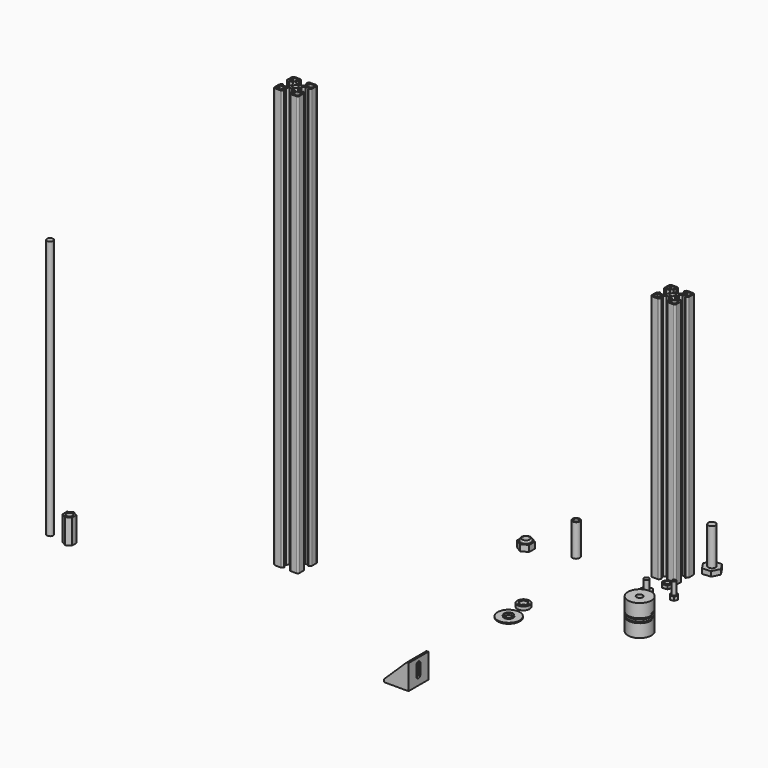
from build123d import *

# Parameters (mm, degrees)
F1_R      = 2.1
F2_DEPTH  = 340
F3_R      = 3
F4_DEPTH  = 34
F5_DEPTH  = 4
F6_R      = 3
F6_R_2    = 2
F7_DEPTH  = 26
F8_R      = 2
F9_DEPTH  = 3
F10_DEPTH = 11
F12_DEPTH = 25
F13_DEPTH = 25
F14_DEPTH = 10.04921
F15_START = 11.79412
F15_DEPTH = 1.02436
F16_START = 13.17687
F16_DEPTH = 1.01812
F17_START = 14.75436
F17_DEPTH = 1.27008
F18_START = 10.61296
F18_DEPTH = 0.97243
F0_R      = 2.1
F20_DEPTH = 200
F21_R     = 2.5
F22_DEPTH = 210
F23_DEPTH = 20
F24_W     = 18.5
F24_H     = 20
F25_DEPTH = 2
F26_W     = 20
F26_H     = 18
F26_H_2   = 2
F27_DEPTH = 1.5
F19_R     = 4
F19_R_2   = 3
F29_DEPTH = 3
F19_R_3   = 5
F19_R_4   = 4.5
F30_DEPTH = 2.8
F31_DEPTH = 0.2
F19_R_5   = 3.75
F19_R_6   = 3.05
F32_DEPTH = 1.5
F19_R_7   = 9
F19_R_8   = 6.5
F33_DEPTH = 0.8
F35_DEPTH = 2
F37_DEPTH = 2
F38_DEPTH = 3
F39_DEPTH = 15
F40_DEPTH = 3
F41_R     = 0.5
F8_R_2    = 1.5
F42_DEPTH = 3
F43_DEPTH = 13
F44_R     = 4.0653248117
F44_R_2   = 3
F45_DEPTH = 5
F46_DEPTH = 7
F47_R     = 1


# Not quite as in the source:
# - ends of sketch curves that miss each other by under 0.0002 mm in the source are joined
# - a feature of the source that left no trace in its solid (it failed there, or was rolled back) is left out


with BuildPart() as f2:
    # F1 (on Top) → F2 (new body)
    with BuildSketch(Plane.XY):
        with BuildLine():
            ThreePointArc((-76.0568475723, -59.3990511647), (-75.9967122677, -59.7013714029), (-75.8254614295, -59.9576660218))
            Line((-75.8254614295, -59.9576660218), (-74.5429985723, -61.2401291647))
            ThreePointArc((-74.5429985723, -61.2401291647), (-74.3297821853, -61.2853778355), (-74.2018372512, -61.1089161811))
            Line((-74.2018372512, -61.1089161811), (-74.2018375723, -60.0487081647))
            Line((-74.2018375723, -60.0487081647), (-71.0852305723, -60.0487081647))
            Line((-71.0852305723, -60.0487081647), (-69.4568475723, -61.6826121647))
            Line((-69.4568475723, -61.6826121647), (-69.4568475723, -63.2678111647))
            Line((-69.4568475723, -63.2678111647), (-69.0759505723, -63.6487081647))
            Line((-69.0759505723, -63.6487081647), (-69.4568475723, -64.0296051647))
            Line((-69.4568475723, -64.0296051647), (-69.4568475723, -65.6148041647))
            Line((-69.4568475723, -65.6148041647), (-71.0852305723, -67.2487081647))
            Line((-71.0852305723, -67.2487081647), (-74.2018375723, -67.2487081647))
            Line((-74.2018375723, -67.2487081647), (-74.2018375723, -66.1885001647))
            ThreePointArc((-74.2018375723, -66.1885001647), (-74.3297821853, -66.0120384939), (-74.5429984286, -66.0572873085))
            Line((-74.5429984286, -66.0572873085), (-75.8254615723, -67.3397501647))
            ThreePointArc((-75.8254615723, -67.3397501647), (-75.9967122677, -67.5960449265), (-76.0568475723, -67.8983651647))
            Line((-76.0568475723, -67.8983651647), (-76.0568475723, -72.2296051647))
            ThreePointArc((-76.0568475723, -72.2296051647), (-75.6261258719, -73.2058338929), (-74.6553495591, -73.6487079596))
            Line((-74.6553495591, -73.6487079596), (-70.0996785723, -73.6487081647))
            ThreePointArc((-70.0996785723, -73.6487081647), (-69.7935318264, -73.5878117907), (-69.5339931474, -73.4143935896))
            Line((-69.5339931474, -73.4143935896), (-68.4300705723, -72.3104711647))
            ThreePointArc((-68.4300705723, -72.3104711647), (-68.3758776892, -72.0380233066), (-68.6068475723, -71.8836941647))
            Line((-68.6068475723, -71.8836941647), (-69.6568475723, -71.8836941647))
            Line((-69.6568475723, -71.8836941647), (-69.6568475723, -68.6836941647))
            Line((-69.6568475723, -68.6836941647), (-68.0622535723, -67.0836941647))
            Line((-68.0622535723, -67.0836941647), (-66.3568475723, -67.0836941647))
            Line((-66.3568475723, -67.0836941647), (-66.0568475723, -66.8237411647))
            Line((-66.0568475723, -66.8237411647), (-65.7568475723, -67.0836941647))
            Line((-65.7568475723, -67.0836941647), (-64.0514415723, -67.0836941647))
            Line((-64.0514415723, -67.0836941647), (-62.4568475723, -68.6836941647))
            Line((-62.4568475723, -68.6836941647), (-62.4568475723, -71.8836941647))
            Line((-62.4568475723, -71.8836941647), (-63.5068475723, -71.8836941647))
            ThreePointArc((-63.5068475723, -71.8836941647), (-63.7378174555, -72.0380233066), (-63.6836242676, -72.31047086))
            Line((-63.6836242676, -72.31047086), (-62.5797015723, -73.4143931647))
            ThreePointArc((-62.5797015723, -73.4143931647), (-62.3201633182, -73.5878117907), (-62.0140165723, -73.6487081647))
            Line((-62.0140165723, -73.6487081647), (-57.4583455723, -73.6487081647))
            ThreePointArc((-57.4583455723, -73.6487081647), (-56.4875692727, -73.2058338929), (-56.0568470783, -72.2296051903))
            Line((-56.0568470783, -72.2296051903), (-56.0568475723, -67.8983651647))
            ThreePointArc((-56.0568475723, -67.8983651647), (-56.1169828769, -67.5960449265), (-56.2882337152, -67.3397503076))
            Line((-56.2882337152, -67.3397503076), (-57.5706965723, -66.0572871647))
            ThreePointArc((-57.5706965723, -66.0572871647), (-57.7839129594, -66.0120384939), (-57.9118578934, -66.1885001483))
            Line((-57.9118578934, -66.1885001483), (-57.9118575723, -67.2487081647))
            Line((-57.9118575723, -67.2487081647), (-61.0284645723, -67.2487081647))
            Line((-61.0284645723, -67.2487081647), (-62.6568475723, -65.6148041647))
            Line((-62.6568475723, -65.6148041647), (-62.6568475723, -64.0296051647))
            Line((-62.6568475723, -64.0296051647), (-63.0377445723, -63.6487081647))
            Line((-63.0377445723, -63.6487081647), (-62.6568475723, -63.2678111647))
            Line((-62.6568475723, -63.2678111647), (-62.6568475723, -61.6826121647))
            Line((-62.6568475723, -61.6826121647), (-61.0284645723, -60.0487081647))
            Line((-61.0284645723, -60.0487081647), (-57.9118575723, -60.0487081647))
            Line((-57.9118575723, -60.0487081647), (-57.9118575723, -61.1089161647))
            ThreePointArc((-57.9118575723, -61.1089161647), (-57.7839129594, -61.2853778355), (-57.5706967161, -61.2401290209))
            Line((-57.5706967161, -61.2401290209), (-56.2882335723, -59.9576661647))
            ThreePointArc((-56.2882335723, -59.9576661647), (-56.1169828769, -59.7013714029), (-56.0568475723, -59.3990511647))
            Line((-56.0568475723, -59.3990511647), (-56.0568475723, -55.0678111647))
            ThreePointArc((-56.0568475723, -55.0678111647), (-56.4875692727, -54.0915824365), (-57.4583455855, -53.6487083698))
            Line((-57.4583455855, -53.6487083698), (-62.0140165723, -53.6487081647))
            ThreePointArc((-62.0140165723, -53.6487081647), (-62.3201633182, -53.7096045387), (-62.5797019973, -53.8830227397))
            Line((-62.5797019973, -53.8830227397), (-63.6836245723, -54.9869451647))
            ThreePointArc((-63.6836245723, -54.9869451647), (-63.7378174555, -55.2593930228), (-63.5068475723, -55.4137221647))
            Line((-63.5068475723, -55.4137221647), (-62.4568475723, -55.4137221647))
            Line((-62.4568475723, -55.4137221647), (-62.4568475723, -58.6137221647))
            Line((-62.4568475723, -58.6137221647), (-64.0514415723, -60.2137221647))
            Line((-64.0514415723, -60.2137221647), (-65.7568475723, -60.2137221647))
            Line((-65.7568475723, -60.2137221647), (-66.0568475723, -60.4736751647))
            Line((-66.0568475723, -60.4736751647), (-66.3568475723, -60.2137221647))
            Line((-66.3568475723, -60.2137221647), (-68.0622535723, -60.2137221647))
            Line((-68.0622535723, -60.2137221647), (-69.6568475723, -58.6137221647))
            Line((-69.6568475723, -58.6137221647), (-69.6568475723, -55.4137221647))
            Line((-69.6568475723, -55.4137221647), (-68.6068475723, -55.4137221647))
            ThreePointArc((-68.6068475723, -55.4137221647), (-68.3758776892, -55.2593930228), (-68.430070877, -54.9869454694))
            Line((-68.430070877, -54.9869454694), (-69.5339935723, -53.8830231647))
            ThreePointArc((-69.5339935723, -53.8830231647), (-69.7935318264, -53.7096045387), (-70.0996785723, -53.6487081647))
            Line((-70.0996785723, -53.6487081647), (-74.6553495723, -53.6487081647))
            ThreePointArc((-74.6553495723, -53.6487081647), (-75.6261258719, -54.0915824365), (-76.0568480663, -55.067811139))
            Line((-76.0568480663, -55.067811139), (-76.0568475723, -59.3990511647))
        make_face()
        with BuildLine():
            Line((-74.8568475723, -72.0296051647), (-74.8568475723, -69.0296051647))
            ThreePointArc((-74.8568475723, -69.0296051647), (-74.7726451834, -68.6531880416), (-74.4455855613, -68.4487082319))
            Line((-74.4455855613, -68.4487082319), (-71.4455855723, -68.4487081647))
            ThreePointArc((-71.4455855723, -68.4487081647), (-70.9974332481, -68.5832975965), (-70.8568471738, -69.0296052379))
            Line((-70.8568471738, -69.0296052379), (-70.8568475723, -72.0296051647))
            ThreePointArc((-70.8568475723, -72.0296051647), (-71.0651110441, -72.369091567), (-71.4553494884, -72.4487077678))
            Line((-71.4553494884, -72.4487077678), (-74.4553495723, -72.4487081647))
            ThreePointArc((-74.4553495723, -72.4487081647), (-74.7231318194, -72.303374032), (-74.8568475723, -72.0296051647))
        make_face(mode=Mode.SUBTRACT)
        with BuildLine():
            ThreePointArc((-61.2568479709, -69.0296052379), (-61.1162618966, -68.5832975965), (-60.6681095129, -68.4487078641))
            Line((-60.6681095129, -68.4487078641), (-57.6681095723, -68.4487081647))
            ThreePointArc((-57.6681095723, -68.4487081647), (-57.3410499613, -68.6531880416), (-57.2568472544, -69.0296052212))
            Line((-57.2568472544, -69.0296052212), (-57.2568475723, -72.0296051647))
            ThreePointArc((-57.2568475723, -72.0296051647), (-57.3905633252, -72.303374032), (-57.6583455515, -72.4487082745))
            Line((-57.6583455515, -72.4487082745), (-60.6583455723, -72.4487081647))
            ThreePointArc((-60.6583455723, -72.4487081647), (-61.0485841005, -72.369091567), (-61.2568478588, -72.0296052052))
            Line((-61.2568478588, -72.0296052052), (-61.2568479709, -69.0296052379))
        make_face(mode=Mode.SUBTRACT)
        with BuildLine():
            ThreePointArc((-70.8568471738, -58.2678110914), (-70.9974332481, -58.7141187328), (-71.4455856318, -58.8487084653))
            Line((-71.4455856318, -58.8487084653), (-74.4455855723, -58.8487081647))
            ThreePointArc((-74.4455855723, -58.8487081647), (-74.7726451834, -58.6442282878), (-74.8568478902, -58.2678111082))
            Line((-74.8568478902, -58.2678111082), (-74.8568475723, -55.2678111647))
            ThreePointArc((-74.8568475723, -55.2678111647), (-74.7231318194, -54.9940422974), (-74.4553495932, -54.8487080549))
            Line((-74.4553495932, -54.8487080549), (-71.4553495723, -54.8487081647))
            ThreePointArc((-71.4553495723, -54.8487081647), (-71.0651110441, -54.9283247624), (-70.8568472858, -55.2678111241))
            Line((-70.8568472858, -55.2678111241), (-70.8568471738, -58.2678110914))
        make_face(mode=Mode.SUBTRACT)
        with Locations((-66.0568475723, -63.6487081647)):
            Circle(F1_R, mode=Mode.SUBTRACT)
        with BuildLine():
            Line((-57.2568475723, -55.2678111647), (-57.2568475723, -58.2678111647))
            ThreePointArc((-57.2568475723, -58.2678111647), (-57.3410499613, -58.6442282878), (-57.6681095834, -58.8487080975))
            Line((-57.6681095834, -58.8487080975), (-60.6681095723, -58.8487081647))
            ThreePointArc((-60.6681095723, -58.8487081647), (-61.1162618966, -58.7141187328), (-61.2568479709, -58.2678110914))
            Line((-61.2568479709, -58.2678110914), (-61.2568475723, -55.2678111647))
            ThreePointArc((-61.2568475723, -55.2678111647), (-61.0485841005, -54.9283247624), (-60.6583456563, -54.8487085616))
            Line((-60.6583456563, -54.8487085616), (-57.6583455723, -54.8487081647))
            ThreePointArc((-57.6583455723, -54.8487081647), (-57.3905633252, -54.9940422974), (-57.2568475723, -55.2678111647))
        make_face(mode=Mode.SUBTRACT)
    extrude(amount=F2_DEPTH)


with BuildPart() as f4:
    # F3 (on Top) → F4 (new body)
    with BuildSketch(Plane.XY):
        with Locations((146.5152157585, 92.1373871341)):
            Circle(F3_R)
    extrude(amount=F4_DEPTH)

    # F3 (on Top) → F5 (join)
    with BuildSketch(Plane.XY):
        Polygon((150.3230751277, 86.3494507985), (153.4316453452, 92.5411219141), (149.623785976, 98.3290582496), (142.7073563893, 97.9253234697), (139.5987861718, 91.7336523541), (143.406645541, 85.9457160186), align=None)
        with Locations((146.5152157585, 92.1373871341)):
            Circle(F3_R, mode=Mode.SUBTRACT)
    extrude(amount=F5_DEPTH)


with BuildPart() as f7:
    # F6 (on Top) → F7 (new body)
    with BuildSketch(Plane.XY):
        with Locations((66.5140599012, 54.7340773046)):
            Circle(F6_R)
        with Locations((66.5140599012, 54.7340773046)):
            Circle(F6_R_2, mode=Mode.SUBTRACT)
    extrude(amount=F7_DEPTH)


with BuildPart() as f9:
    # F8 (on Top) → F9 (new body)
    with BuildSketch(Plane.XY):
        Polygon((135.9405546962, 38.4316313278), (138.0129348412, 42.5594120715), (135.4743619284, 46.4180362952), (130.8634088706, 46.1488797752), (128.7910287256, 42.0210990315), (131.3296016384, 38.1624748078), align=None)
        with Locations((133.4019817834, 42.2902555515)):
            Circle(F8_R, mode=Mode.SUBTRACT)
    extrude(amount=F9_DEPTH)

    # F8 (on Top) → F10 (join)
    with BuildSketch(Plane.XY):
        with Locations((133.4019817834, 42.2902555515)):
            Circle(F8_R)
    extrude(amount=F10_DEPTH)


with BuildPart() as f12:
    # F11 (on Top) → F12 (new body)
    with BuildSketch(Plane.XY):
        with BuildLine():
            Line((164.1954952478, 0), (165.6954952478, 0))
            ThreePointArc((165.6954952478, 0), (161.6954952478, 4), (157.6954952478, 0))
            Line((157.6954952478, 0), (159.1954952478, 0))
            ThreePointArc((159.1954952478, 0), (161.6954952478, 2.5), (164.1954952478, 0))
        make_face()
        with BuildLine():
            ThreePointArc((157.6954952478, 0), (161.6954952478, -4), (165.6954952478, 0))
            Line((165.6954952478, 0), (164.1954952478, 0))
            ThreePointArc((164.1954952478, 0), (161.6954952478, -2.5), (159.1954952478, 0))
            Line((159.1954952478, 0), (157.6954952478, 0))
        make_face()
        with BuildLine():
            Line((161.6954952478, 0), (164.1954952478, 0))
            ThreePointArc((164.1954952478, 0), (161.6954952478, 2.5), (159.1954952478, 0))
            Line((159.1954952478, 0), (161.6954952478, 0))
        make_face()
        with BuildLine():
            ThreePointArc((159.1954952478, 0), (161.6954952478, -2.5), (164.1954952478, 0))
            Line((164.1954952478, 0), (161.6954952478, 0))
            Line((161.6954952478, 0), (159.1954952478, 0))
        make_face()
        with BuildLine():
            ThreePointArc((157.6954952478, 0), (161.6954952478, 4), (165.6954952478, 0))
            Line((165.6954952478, 0), (171.1954952478, 0))
            ThreePointArc((171.1954952478, 0), (161.6954952478, 9.5), (152.1954952478, 0))
            Line((152.1954952478, 0), (157.6954952478, 0))
        make_face()
        with BuildLine():
            Line((171.1954952478, 0), (165.6954952478, 0))
            ThreePointArc((165.6954952478, 0), (161.6954952478, -4), (157.6954952478, 0))
            Line((157.6954952478, 0), (152.1954952478, 0))
            ThreePointArc((152.1954952478, 0), (161.6954952478, -9.5), (171.1954952478, 0))
        make_face()
    extrude(amount=F12_DEPTH)

    # F11 (on Top) → F13 (cut)
    with BuildSketch(Plane.XY):
        with BuildLine():
            Line((161.6954952478, 0), (164.1954952478, 0))
            ThreePointArc((164.1954952478, 0), (161.6954952478, 2.5), (159.1954952478, 0))
            Line((159.1954952478, 0), (161.6954952478, 0))
        make_face()
        with BuildLine():
            ThreePointArc((159.1954952478, 0), (161.6954952478, -2.5), (164.1954952478, 0))
            Line((164.1954952478, 0), (161.6954952478, 0))
            Line((161.6954952478, 0), (159.1954952478, 0))
        make_face()
    extrude(amount=F13_DEPTH, mode=Mode.SUBTRACT)

    # F11 (on Top) → F14 (cut)
    with BuildSketch(Plane.XY):
        with BuildLine():
            Line((164.1954952478, 0), (165.6954952478, 0))
            ThreePointArc((165.6954952478, 0), (161.6954952478, 4), (157.6954952478, 0))
            Line((157.6954952478, 0), (159.1954952478, 0))
            ThreePointArc((159.1954952478, 0), (161.6954952478, 2.5), (164.1954952478, 0))
        make_face()
        with BuildLine():
            ThreePointArc((157.6954952478, 0), (161.6954952478, -4), (165.6954952478, 0))
            Line((165.6954952478, 0), (164.1954952478, 0))
            ThreePointArc((164.1954952478, 0), (161.6954952478, -2.5), (159.1954952478, 0))
            Line((159.1954952478, 0), (157.6954952478, 0))
        make_face()
    extrude(amount=F14_DEPTH, mode=Mode.SUBTRACT)

    # F11 (on Top) → F15 (cut)
    with BuildSketch(Plane.XY.offset(F15_START)):
        with BuildLine():
            ThreePointArc((157.6954952478, 0), (161.6954952478, 4), (165.6954952478, 0))
            Line((165.6954952478, 0), (171.1954952478, 0))
            ThreePointArc((171.1954952478, 0), (161.6954952478, 9.5), (152.1954952478, 0))
            Line((152.1954952478, 0), (157.6954952478, 0))
        make_face()
    extrude(amount=F15_DEPTH, mode=Mode.SUBTRACT)

    # F11 (on Top) → F16 (cut)
    with BuildSketch(Plane.XY.offset(F16_START)):
        with BuildLine():
            Line((171.1954952478, 0), (165.6954952478, 0))
            ThreePointArc((165.6954952478, 0), (161.6954952478, -4), (157.6954952478, 0))
            Line((157.6954952478, 0), (152.1954952478, 0))
            ThreePointArc((152.1954952478, 0), (161.6954952478, -9.5), (171.1954952478, 0))
        make_face()
    extrude(amount=F16_DEPTH, mode=Mode.SUBTRACT)

    # F11 (on Top) → F17 (cut)
    with BuildSketch(Plane.XY.offset(F17_START)):
        with BuildLine():
            ThreePointArc((157.6954952478, 0), (161.6954952478, 4), (165.6954952478, 0))
            Line((165.6954952478, 0), (171.1954952478, 0))
            ThreePointArc((171.1954952478, 0), (161.6954952478, 9.5), (152.1954952478, 0))
            Line((152.1954952478, 0), (157.6954952478, 0))
        make_face()
    extrude(amount=F17_DEPTH, mode=Mode.SUBTRACT)

    # F11 (on Top) → F18 (cut)
    with BuildSketch(Plane.XY.offset(F18_START)):
        with BuildLine():
            Line((171.1954952478, 0), (165.6954952478, 0))
            ThreePointArc((165.6954952478, 0), (161.6954952478, -4), (157.6954952478, 0))
            Line((157.6954952478, 0), (152.1954952478, 0))
            ThreePointArc((152.1954952478, 0), (161.6954952478, -9.5), (171.1954952478, 0))
        make_face()
    extrude(amount=F18_DEPTH, mode=Mode.SUBTRACT)


with BuildPart() as f20:
    # F0 (on Top) → F20 (new body)
    with BuildSketch(Plane.XY):
        with BuildLine():
            ThreePointArc((121.536751085, 82.7884841895), (120.5659747722, 82.3456101228), (120.1352525778, 81.3693814202))
            Line((120.1352525778, 81.3693814202), (120.1352530718, 77.0381413946))
            ThreePointArc((120.1352530718, 77.0381413946), (120.1953883764, 76.7358211563), (120.3666392146, 76.4795265374))
            Line((120.3666392146, 76.4795265374), (121.6491020718, 75.1970633946))
            ThreePointArc((121.6491020718, 75.1970633946), (121.8623184588, 75.1518147238), (121.9902633929, 75.3282763781))
            Line((121.9902633929, 75.3282763781), (121.9902630718, 76.3884843946))
            Line((121.9902630718, 76.3884843946), (125.1068700718, 76.3884843946))
            Line((125.1068700718, 76.3884843946), (126.7352530718, 74.7545803946))
            Line((126.7352530718, 74.7545803946), (126.7352530718, 73.1693813946))
            Line((126.7352530718, 73.1693813946), (127.1161500718, 72.7884843946))
            Line((127.1161500718, 72.7884843946), (126.7352530718, 72.4075873946))
            Line((126.7352530718, 72.4075873946), (126.7352530718, 70.8223883946))
            Line((126.7352530718, 70.8223883946), (125.1068700718, 69.1884843946))
            Line((125.1068700718, 69.1884843946), (121.9902630718, 69.1884843946))
            Line((121.9902630718, 69.1884843946), (121.9902630718, 70.2486923946))
            ThreePointArc((121.9902630718, 70.2486923946), (121.8623184588, 70.4251540653), (121.6491022155, 70.3799052508))
            Line((121.6491022155, 70.3799052508), (120.3666390718, 69.0974423946))
            ThreePointArc((120.3666390718, 69.0974423946), (120.1953883764, 68.8411476328), (120.1352530718, 68.5388273946))
            Line((120.1352530718, 68.5388273946), (120.1352530718, 64.2075873946))
            ThreePointArc((120.1352530718, 64.2075873946), (120.5659747722, 63.2313586663), (121.536751085, 62.7884845996))
            Line((121.536751085, 62.7884845996), (126.0924220718, 62.7884843946))
            ThreePointArc((126.0924220718, 62.7884843946), (126.3985688177, 62.8493807685), (126.6581074967, 63.0227989696))
            Line((126.6581074967, 63.0227989696), (127.7620300718, 64.1267213946))
            ThreePointArc((127.7620300718, 64.1267213946), (127.8162229549, 64.3991692526), (127.5852530718, 64.5534983946))
            Line((127.5852530718, 64.5534983946), (126.5352530718, 64.5534983946))
            Line((126.5352530718, 64.5534983946), (126.5352530718, 67.7534983946))
            Line((126.5352530718, 67.7534983946), (128.1298470718, 69.3534983946))
            Line((128.1298470718, 69.3534983946), (129.8352530718, 69.3534983946))
            Line((129.8352530718, 69.3534983946), (130.1352530718, 69.6134513946))
            Line((130.1352530718, 69.6134513946), (130.4352530718, 69.3534983946))
            Line((130.4352530718, 69.3534983946), (132.1406590718, 69.3534983946))
            Line((132.1406590718, 69.3534983946), (133.7352530718, 67.7534983946))
            Line((133.7352530718, 67.7534983946), (133.7352530718, 64.5534983946))
            Line((133.7352530718, 64.5534983946), (132.6852530718, 64.5534983946))
            ThreePointArc((132.6852530718, 64.5534983946), (132.4542831887, 64.3991692526), (132.5084763765, 64.1267216993))
            Line((132.5084763765, 64.1267216993), (133.6123990718, 63.0227993946))
            ThreePointArc((133.6123990718, 63.0227993946), (133.8719373259, 62.8493807685), (134.1780840718, 62.7884843946))
            Line((134.1780840718, 62.7884843946), (138.7337550718, 62.7884843946))
            ThreePointArc((138.7337550718, 62.7884843946), (139.7045313714, 63.2313586663), (140.1352535658, 64.2075873689))
            Line((140.1352535658, 64.2075873689), (140.1352530718, 68.5388273946))
            ThreePointArc((140.1352530718, 68.5388273946), (140.0751177672, 68.8411476328), (139.9038669289, 69.0974422517))
            Line((139.9038669289, 69.0974422517), (138.6214040718, 70.3799053946))
            ThreePointArc((138.6214040718, 70.3799053946), (138.4081876847, 70.4251540653), (138.2802427507, 70.248692411))
            Line((138.2802427507, 70.248692411), (138.2802430718, 69.1884843946))
            Line((138.2802430718, 69.1884843946), (135.1636360718, 69.1884843946))
            Line((135.1636360718, 69.1884843946), (133.5352530718, 70.8223883946))
            Line((133.5352530718, 70.8223883946), (133.5352530718, 72.4075873946))
            Line((133.5352530718, 72.4075873946), (133.1543560718, 72.7884843946))
            Line((133.1543560718, 72.7884843946), (133.5352530718, 73.1693813946))
            Line((133.5352530718, 73.1693813946), (133.5352530718, 74.7545803946))
            Line((133.5352530718, 74.7545803946), (135.1636360718, 76.3884843946))
            Line((135.1636360718, 76.3884843946), (138.2802430718, 76.3884843946))
            Line((138.2802430718, 76.3884843946), (138.2802430718, 75.3282763946))
            ThreePointArc((138.2802430718, 75.3282763946), (138.4081876847, 75.1518147238), (138.621403928, 75.1970635383))
            Line((138.621403928, 75.1970635383), (139.9038670718, 76.4795263946))
            ThreePointArc((139.9038670718, 76.4795263946), (140.0751177672, 76.7358211563), (140.1352530718, 77.0381413946))
            Line((140.1352530718, 77.0381413946), (140.1352530718, 81.3693813946))
            ThreePointArc((140.1352530718, 81.3693813946), (139.7045313714, 82.3456101228), (138.7337550586, 82.7884841895))
            Line((138.7337550586, 82.7884841895), (134.1780840718, 82.7884843946))
            ThreePointArc((134.1780840718, 82.7884843946), (133.8719373259, 82.7275880206), (133.6123986468, 82.5541698195))
            Line((133.6123986468, 82.5541698195), (132.5084760718, 81.4502473946))
            ThreePointArc((132.5084760718, 81.4502473946), (132.4542831887, 81.1777995365), (132.6852530718, 81.0234703946))
            Line((132.6852530718, 81.0234703946), (133.7352530718, 81.0234703946))
            Line((133.7352530718, 81.0234703946), (133.7352530718, 77.8234703946))
            Line((133.7352530718, 77.8234703946), (132.1406590718, 76.2234703946))
            Line((132.1406590718, 76.2234703946), (130.4352530718, 76.2234703946))
            Line((130.4352530718, 76.2234703946), (130.1352530718, 75.9635173946))
            Line((130.1352530718, 75.9635173946), (129.8352530718, 76.2234703946))
            Line((129.8352530718, 76.2234703946), (128.1298470718, 76.2234703946))
            Line((128.1298470718, 76.2234703946), (126.5352530718, 77.8234703946))
            Line((126.5352530718, 77.8234703946), (126.5352530718, 81.0234703946))
            Line((126.5352530718, 81.0234703946), (127.5852530718, 81.0234703946))
            ThreePointArc((127.5852530718, 81.0234703946), (127.8162229549, 81.1777995365), (127.7620297671, 81.4502470898))
            Line((127.7620297671, 81.4502470898), (126.6581070718, 82.5541693946))
            ThreePointArc((126.6581070718, 82.5541693946), (126.3985688177, 82.7275880206), (126.0924220718, 82.7884843946))
            Line((126.0924220718, 82.7884843946), (121.536751085, 82.7884841895))
        make_face()
        with BuildLine():
            Line((124.7367510718, 63.9884843946), (121.7367510718, 63.9884843946))
            ThreePointArc((121.7367510718, 63.9884843946), (121.4689688247, 64.1338185272), (121.3352527124, 64.4075873422))
            Line((121.3352527124, 64.4075873422), (121.3352530718, 67.4075873946))
            ThreePointArc((121.3352530718, 67.4075873946), (121.4194554607, 67.7840045177), (121.7465150828, 67.9884843273))
            Line((121.7465150828, 67.9884843273), (124.7465150718, 67.9884843946))
            ThreePointArc((124.7465150718, 67.9884843946), (125.194667396, 67.8538949627), (125.3352534703, 67.4075873213))
            Line((125.3352534703, 67.4075873213), (125.3352530718, 64.4075873946))
            ThreePointArc((125.3352530718, 64.4075873946), (125.1269896, 64.0681009923), (124.7367510718, 63.9884843946))
        make_face(mode=Mode.SUBTRACT)
        with BuildLine():
            ThreePointArc((134.9352526732, 67.4075873213), (135.0758387476, 67.8538949627), (135.5239911312, 67.9884846952))
            Line((135.5239911312, 67.9884846952), (138.5239910718, 67.9884843946))
            ThreePointArc((138.5239910718, 67.9884843946), (138.8510506828, 67.7840045177), (138.9352533897, 67.407587338))
            Line((138.9352533897, 67.407587338), (138.9352530718, 64.4075873946))
            ThreePointArc((138.9352530718, 64.4075873946), (138.8015373189, 64.1338185272), (138.5337550926, 63.9884842848))
            Line((138.5337550926, 63.9884842848), (135.5337550718, 63.9884843946))
            ThreePointArc((135.5337550718, 63.9884843946), (135.1435165436, 64.0681009923), (134.9352527853, 64.407587354))
            Line((134.9352527853, 64.407587354), (134.9352526732, 67.4075873213))
        make_face(mode=Mode.SUBTRACT)
        with Locations((130.1352530718, 72.7884843946)):
            Circle(F0_R, mode=Mode.SUBTRACT)
        with BuildLine():
            ThreePointArc((121.3352527124, 81.1693814469), (121.4689688247, 81.4431502619), (121.7367510509, 81.5884845043))
            Line((121.7367510509, 81.5884845043), (124.7367510718, 81.5884843946))
            ThreePointArc((124.7367510718, 81.5884843946), (125.1269896, 81.5088677968), (125.3352533583, 81.1693814351))
            Line((125.3352533583, 81.1693814351), (125.3352530718, 78.1693813946))
            ThreePointArc((125.3352530718, 78.1693813946), (125.194667396, 77.7230738264), (124.7465150123, 77.5884840939))
            Line((124.7465150123, 77.5884840939), (121.7465150718, 77.5884843946))
            ThreePointArc((121.7465150718, 77.5884843946), (121.4194554607, 77.7929642714), (121.3352527539, 78.1693814511))
            Line((121.3352527539, 78.1693814511), (121.3352527124, 81.1693814469))
        make_face(mode=Mode.SUBTRACT)
        with BuildLine():
            Line((135.5337550718, 81.5884843946), (138.5337550718, 81.5884843946))
            ThreePointArc((138.5337550718, 81.5884843946), (138.8015373189, 81.4431502619), (138.9352534311, 81.1693814469))
            Line((138.9352534311, 81.1693814469), (138.9352530718, 78.1693813946))
            ThreePointArc((138.9352530718, 78.1693813946), (138.8510506828, 77.7929642714), (138.5239910607, 77.5884844618))
            Line((138.5239910607, 77.5884844618), (135.5239910718, 77.5884843946))
            ThreePointArc((135.5239910718, 77.5884843946), (135.0758387476, 77.7230738264), (134.9352526732, 78.1693814678))
            Line((134.9352526732, 78.1693814678), (134.9352530718, 81.1693813946))
            ThreePointArc((134.9352530718, 81.1693813946), (135.1435165436, 81.5088677968), (135.5337550718, 81.5884843946))
        make_face(mode=Mode.SUBTRACT)
    extrude(amount=F20_DEPTH)


with BuildPart() as f22:
    # F21 (on Top) → F22 (new body)
    with BuildSketch(Plane.XY):
        with Locations((-212.2113704681, -129.4149756432)):
            Circle(F21_R)
    extrude(amount=F22_DEPTH)


with BuildPart() as f23:
    # F21 (on Top) → F23 (new body)
    with BuildSketch(Plane.XY):
        Polygon((-191.757559632, -128.4082318926), (-195.5637412817, -126.2107318926), (-199.3699229313, -128.4082318926), (-199.3699229313, -132.8032318926), (-195.5637412817, -135.0007318926), (-191.757559632, -132.8032318926), align=None)
        with Locations((-195.5637412817, -130.6057318926)):
            Circle(F21_R, mode=Mode.SUBTRACT)
    extrude(amount=F23_DEPTH)


with BuildPart() as f25:
    # F24 (on Top) → F25 (new body)
    with BuildSketch(Plane.XY):
        with Locations((88.1310835183, -145.4428576239)):
            Rectangle(F24_W, F24_H)
        with BuildLine():
            ThreePointArc((83.4745168698, -147.4428576239), (81.4746621909, -145.4187481227), (83.5227323685, -143.4434388919))
            Line((83.5227323685, -143.4434388919), (92.7875246899, -143.4428576278))
            ThreePointArc((92.7875246899, -143.4428576278), (94.2018193664, -144.028599699), (94.7876501679, -145.4428576239))
            ThreePointArc((94.7876501679, -145.4428576239), (94.2018109334, -146.8571239812), (92.7875008386, -147.4428576183))
            Line((92.7875008386, -147.4428576183), (83.4745168698, -147.4428576239))
        make_face(mode=Mode.SUBTRACT)
    extrude(amount=F25_DEPTH)

    # F26 (on face) → F27 (join)
    with BuildSketch(Plane.YZ.offset(97.3810835183)):
        with Locations((-145.4428576239, 11)):
            Rectangle(F26_W, F26_H)
        with BuildLine():
            ThreePointArc((-147.4428576239, 15.2325471863), (-145.4428576239, 17.2325471863), (-143.4428576239, 15.2325471863))
            Line((-143.4428576239, 15.2325471863), (-143.4428576239, 6.9971131161))
            ThreePointArc((-143.4428576239, 6.9971131161), (-145.4428576239, 4.9971131161), (-147.4428576239, 6.9971131161))
            Line((-147.4428576239, 6.9971131161), (-147.4428576239, 15.2325471863))
        make_face(mode=Mode.SUBTRACT)
        with Locations((-145.4428576239, 1)):
            Rectangle(F26_W, F26_H_2)
    extrude(amount=F27_DEPTH)

    # F34 (on face) → F35 (join)
    with BuildSketch(Plane.XZ.offset(155.4428576239)):
        Polygon((97.3810835183, 20), (78.8810835183, 2), (97.3810835183, 2), align=None)
    extrude(amount=-F35_DEPTH)

    # F36 (on face) → F37 (join)
    with BuildSketch(Plane(origin=(0, -135.4428576239, 0), x_dir=(-1, 0, 0), z_dir=(0, 1, 0))):
        Polygon((-78.8810835183, 2), (-97.3810835183, 20), (-97.3810835183, 2), align=None)
    extrude(amount=-F37_DEPTH)


with BuildPart() as f29:
    # F19 (on Top) → F29 (new body)
    with BuildSketch(Plane.XY):
        with Locations((83.691842854, -20.0953492895)):
            Circle(F19_R)
        with Locations((83.691842854, -20.0953492895)):
            Circle(F19_R_2, mode=Mode.SUBTRACT)
    extrude(amount=F29_DEPTH)



with BuildPart() as f29b:
    # F19 (on Top) → F29, piece 2 (new body)
    with BuildSketch(Plane.XY):
        with Locations((83.691842854, -20.0953492895)):
            Circle(F19_R_3)
        with Locations((83.691842854, -20.0953492895)):
            Circle(F19_R_4, mode=Mode.SUBTRACT)
    extrude(amount=F29_DEPTH)


with BuildPart() as f29_1:
    add(f29.part)

    add(f29b.part)  # F30 merges F29b
    # F19 (on Top) → F30 (join)
    with BuildSketch(Plane.XY):
        with Locations((83.691842854, -20.0953492895)):
            Circle(F19_R_4)
        with Locations((83.691842854, -20.0953492895)):
            Circle(F19_R, mode=Mode.SUBTRACT)
    extrude(amount=F30_DEPTH)

    # F31 (cut): a face of the model
    f31_faces = [f29_1.faces().sort_by_distance(p)[0] for p in [
        (78.8332642103, -20.0953492895, 0),
    ]]
    extrude(f31_faces, amount=-F31_DEPTH, mode=Mode.SUBTRACT)


with BuildPart() as f32:
    # F19 (on Top) → F32 (new body)
    with BuildSketch(Plane.XY):
        with Locations((85.1471349597, -36.9014516473)):
            Circle(F19_R_5)
        with Locations((85.1471349597, -36.9014516473)):
            Circle(F19_R_6, mode=Mode.SUBTRACT)
    extrude(amount=F32_DEPTH)

    # F19 (on Top) → F33 (join)
    with BuildSketch(Plane.XY):
        with Locations((85.1471349597, -36.9014516473)):
            Circle(F19_R_7)
        with Locations((85.1471349597, -36.9014516473)):
            Circle(F19_R_8, mode=Mode.SUBTRACT)
        with Locations((85.1471349597, -36.9014516473)):
            Circle(F19_R_8)
        with Locations((85.1471349597, -36.9014516473)):
            Circle(F19_R_5, mode=Mode.SUBTRACT)
    extrude(amount=F33_DEPTH)


with BuildPart() as f38:
    # F8 (on Top) → F38 (new body)
    with BuildSketch(Plane.XY):
        Polygon((135.9405546962, 38.4316313278), (138.0129348412, 42.5594120715), (135.4743619284, 46.4180362952), (130.8634088706, 46.1488797752), (128.7910287256, 42.0210990315), (131.3296016384, 38.1624748078), align=None)
        with Locations((133.4019817834, 42.2902555515)):
            Circle(F8_R, mode=Mode.SUBTRACT)
    extrude(amount=-F38_DEPTH)

    # F8 (on Top) → F39 (join)
    with BuildSketch(Plane.XY):
        with Locations((133.4019817834, 42.2902555515)):
            Circle(F8_R)
    extrude(amount=-F39_DEPTH)


with BuildPart() as f40:
    # F8 (on Top) → F40 (new body)
    with BuildSketch(Plane.XY):
        Polygon((141.3886775457, 58.9997099295), (138.9686770966, 62.2365187221), (134.9555182305, 61.7591412522), (133.3623598135, 58.0449549898), (135.7823602626, 54.8081461973), (139.7955191288, 55.2855236671), align=None)
        with Locations((137.3755186796, 58.5223324597)):
            Circle(F8_R, mode=Mode.SUBTRACT)
    extrude(amount=F40_DEPTH)

    # F41
    f41_edges = [f40.edges().sort_by_distance(p)[0] for p in [
        (140.592098, 57.142617, 3),
        (134.57236, 56.426551, 3),
        (134.158939, 59.902048, 3),
        (136.962098, 61.99783, 3),
        (140.178677, 60.618114, 3),
        (137.78894, 55.046835, 3),
        (137.78894, 55.046835, 0),
        (140.592098, 57.142617, 0),
        (140.178677, 60.618114, 0),
        (136.962098, 61.99783, 0),
        (134.158939, 59.902048, 0),
        (134.57236, 56.426551, 0),
        (135.375519, 58.522332, 0),
    ]]
    fillet(f41_edges, radius=F41_R)


with BuildPart() as f42:
    # F8 (on Top) → F42 (new body)
    with BuildSketch(Plane.XY):
        Polygon((152.7251302748, 45.9721328555), (153.8311482479, 48.6386019771), (152.0749272367, 50.9296761996), (149.2126882524, 50.5542813005), (148.1066702793, 47.8878121789), (149.8628912906, 45.5967379564), align=None)
        with Locations((150.9689092636, 48.263207078)):
            Circle(F8_R_2, mode=Mode.SUBTRACT)
        with Locations((150.9689092636, 48.263207078)):
            Circle(F8_R_2)
    extrude(amount=F42_DEPTH)

    # F8 (on Top) → F43 (join)
    with BuildSketch(Plane.XY):
        with Locations((150.9689092636, 48.263207078)):
            Circle(F8_R_2)
    extrude(amount=F43_DEPTH)


with BuildPart() as f45:
    # F44 (on Top) → F45 (new body)
    with BuildSketch(Plane.XY):
        Polygon((34.2440637603, 38.2117694555), (39.3222931422, 40.9585711734), (39.4826077663, 46.7298476834), (34.5646930084, 49.7543224754), (29.4864636265, 47.0075207574), (29.3261490024, 41.2362442475), align=None)
        with Locations((34.4043783844, 43.9830459654)):
            Circle(F44_R, mode=Mode.SUBTRACT)
        with Locations((34.4043783844, 43.9830459654)):
            Circle(F44_R)
        with Locations((34.4043783844, 43.9830459654)):
            Circle(F44_R_2, mode=Mode.SUBTRACT)
    extrude(amount=F45_DEPTH)

    # F44 (on Top) → F46 (join)
    with BuildSketch(Plane.XY):
        with Locations((34.4043783844, 43.9830459654)):
            Circle(F44_R)
        with Locations((34.4043783844, 43.9830459654)):
            Circle(F44_R_2, mode=Mode.SUBTRACT)
    extrude(amount=F46_DEPTH)

    # F47
    f47_edges = [f45.edges().sort_by_distance(p)[0] for p in [
        (30.339054, 43.983046, 7),
    ]]
    fillet(f47_edges, radius=F47_R)


solid = Compound([f2.part, f4.part, f7.part, f9.part, f12.part, f20.part, f22.part, f23.part, f25.part, f29_1.part, f32.part, f38.part, f40.part, f42.part, f45.part])
